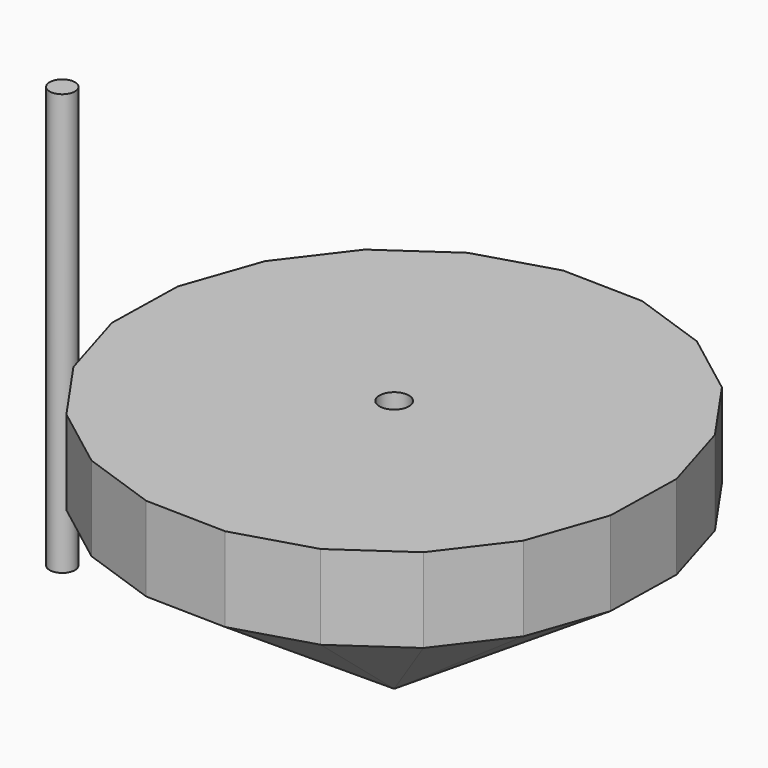
from build123d import *

# Parameters (mm, degrees)
F1_DEPTH     = 30
F2_T1_DEPTH  = 273.0855354784
F2_T3_DEPTH  = 273.0855354784
F2_T5_DEPTH  = 273.0855354784
F2_T7_DEPTH  = 273.0855354784
F2_T9_DEPTH  = 273.0855354784
F2_T11_DEPTH = 273.0855354784
F2_T13_DEPTH = 273.0855354784
F2_T15_DEPTH = 273.0855354784
F2_T17_DEPTH = 273.0855354784
F2_T19_DEPTH = 273.0855354784
F2_T21_DEPTH = 273.0855354784
F2_T23_DEPTH = 273.0855354784
F2_T25_DEPTH = 273.0855354784
F2_T27_DEPTH = 273.0855354784
F2_T29_DEPTH = 273.0855354784
F2_T31_DEPTH = 273.0855354784
F2_T33_DEPTH = 273.0855354784
F2_T35_DEPTH = 273.0855354784
F2_T37_DEPTH = 273.0855354784
F2_T39_DEPTH = 273.0855354784
F3_R         = 1.75
F4_DEPTH     = 24
F5_R         = 1.5
F6_DEPTH     = 50


# Not quite as in the source:
# - a fillet or chamfer that OpenCascade refuses, or shapes differently, is made with other operations: its cross-section is extruded or revolved along the edge and cut away or added


with BuildPart() as f1:
    # F0 (on Top) → F1 (new body)
    with BuildSketch(Plane.XY):
        Polygon((13.2507014279, -27.4548412117), (21.0861784508, -22.0164137096), (26.8575934109, -14.4228662363), (30, -5.4175081257), (30.2057975669, 4.1181534262), (27.4548412117, 13.2507014279), (22.0164137096, 21.0861784508), (14.4228662363, 26.8575934109), (5.4175081257, 30), (-4.1181534262, 30.2057975669), (-13.2507014279, 27.4548412117), (-21.0861784508, 22.0164137096), (-26.8575934109, 14.4228662363), (-30, 5.4175081257), (-30.2057975669, -4.1181534262), (-27.4548412117, -13.2507014279), (-22.0164137096, -21.0861784508), (-14.4228662363, -26.8575934109), (-5.4175081257, -30), (4.1181534262, -30.2057975669), align=None)
    extrude(amount=F1_DEPTH)

    # F2: chamfer of 30 x 20 on 20 edges, made by hand

    # F2_s2 → F2_t1 (cut)
    with BuildSketch(Plane(origin=(-128.9192417481, 44.9861815336, 0), x_dir=(0, 0, 1), z_dir=(0.944167486, -0.3294658683, 0))):
        Polygon((20, 30.1099085987), (0, 0.1099085987), (0, 30.1099085987), align=None)
    extrude(amount=F2_T1_DEPTH, mode=Mode.SUBTRACT)

    # F2_s4 → F2_t3 (cut)
    with BuildSketch(Plane(origin=(-136.5109795463, 2.9461644886, 0), x_dir=(0, 0, 1), z_dir=(0.9997671924, -0.0215768622, 0))):
        Polygon((20, 30.1099085987), (0, 0.1099085987), (0, 30.1099085987), align=None)
    extrude(amount=F2_T3_DEPTH, mode=Mode.SUBTRACT)

    # F2_s6 → F2_t5 (cut)
    with BuildSketch(Plane(origin=(-130.7400715385, -39.3822436636, 0), x_dir=(0, 0, 1), z_dir=(0.9575027202, 0.2884242374, 0))):
        Polygon((20, 30.1099085987), (0, 0.1099085987), (0, 30.1099085987), align=None)
    extrude(amount=F2_T5_DEPTH, mode=Mode.SUBTRACT)

    # F2_s8 → F2_t7 (cut)
    with BuildSketch(Plane(origin=(-39.3822436636, 130.7400715385, 0), x_dir=(0, 0, 1), z_dir=(0.2884242374, -0.9575027202, 0))):
        Polygon((20, 30.1099085987), (0, 0.1099085987), (0, 30.1099085987), align=None)
    extrude(amount=F2_T7_DEPTH, mode=Mode.SUBTRACT)

    # F2_s10 → F2_t9 (cut)
    with BuildSketch(Plane(origin=(-77.8556434138, 112.171414409, 0), x_dir=(0, 0, 1), z_dir=(0.5701923632, -0.8215112105, 0))):
        Polygon((20, 30.1099085987), (0, 0.1099085987), (0, 30.1099085987), align=None)
    extrude(amount=F2_T9_DEPTH, mode=Mode.SUBTRACT)

    # F2_s12 → F2_t11 (cut)
    with BuildSketch(Plane(origin=(-108.7079903345, 82.6226376928, 0), x_dir=(0, 0, 1), z_dir=(0.7961460877, -0.6051044597, 0))):
        Polygon((20, 30.1099085987), (0, 0.1099085987), (0, 30.1099085987), align=None)
    extrude(amount=F2_T11_DEPTH, mode=Mode.SUBTRACT)

    # F2_s14 → F2_t13 (cut)
    with BuildSketch(Plane(origin=(-112.171414409, -77.8556434138, 0), x_dir=(0, 0, 1), z_dir=(0.8215112105, 0.5701923632, 0))):
        Polygon((20, 30.1099085987), (0, 0.1099085987), (0, 30.1099085987), align=None)
    extrude(amount=F2_T13_DEPTH, mode=Mode.SUBTRACT)

    # F2_s16 → F2_t15 (cut)
    with BuildSketch(Plane(origin=(-82.6226376928, -108.7079903345, 0), x_dir=(0, 0, 1), z_dir=(0.6051044597, 0.7961460877, 0))):
        Polygon((20, 30.1099085987), (0, 0.1099085987), (0, 30.1099085987), align=None)
    extrude(amount=F2_T15_DEPTH, mode=Mode.SUBTRACT)

    # F2_s18 → F2_t17 (cut)
    with BuildSketch(Plane(origin=(-44.9861815336, -128.9192417481, 0), x_dir=(0, 0, 1), z_dir=(0.3294658683, 0.944167486, 0))):
        Polygon((20, 30.1099085987), (0, 0.1099085987), (0, 30.1099085987), align=None)
    extrude(amount=F2_T17_DEPTH, mode=Mode.SUBTRACT)

    # F2_s20 → F2_t19 (cut)
    with BuildSketch(Plane(origin=(-2.9461644886, -136.5109795463, 0), x_dir=(0, 0, 1), z_dir=(0.0215768622, 0.9997671924, 0))):
        Polygon((20, 30.1099085987), (0, 0.1099085987), (0, 30.1099085987), align=None)
    extrude(amount=F2_T19_DEPTH, mode=Mode.SUBTRACT)

    # F2_s22 → F2_t21 (cut)
    with BuildSketch(Plane(origin=(39.3822436636, -130.7400715385, 0), x_dir=(0, 0, 1), z_dir=(-0.2884242374, 0.9575027202, 0))):
        Polygon((20, 30.1099085987), (0, 0.1099085987), (0, 30.1099085987), align=None)
    extrude(amount=F2_T21_DEPTH, mode=Mode.SUBTRACT)

    # F2_s24 → F2_t23 (cut)
    with BuildSketch(Plane(origin=(77.8556434138, -112.171414409, 0), x_dir=(0, 0, 1), z_dir=(-0.5701923632, 0.8215112105, 0))):
        Polygon((20, 30.1099085987), (0, 0.1099085987), (0, 30.1099085987), align=None)
    extrude(amount=F2_T23_DEPTH, mode=Mode.SUBTRACT)

    # F2_s26 → F2_t25 (cut)
    with BuildSketch(Plane(origin=(108.7079903345, -82.6226376928, 0), x_dir=(0, 0, 1), z_dir=(-0.7961460877, 0.6051044597, 0))):
        Polygon((20, 30.1099085987), (0, 0.1099085987), (0, 30.1099085987), align=None)
    extrude(amount=F2_T25_DEPTH, mode=Mode.SUBTRACT)

    # F2_s28 → F2_t27 (cut)
    with BuildSketch(Plane(origin=(128.9192417481, -44.9861815336, 0), x_dir=(0, 0, 1), z_dir=(-0.944167486, 0.3294658683, 0))):
        Polygon((20, 30.1099085987), (0, 0.1099085987), (0, 30.1099085987), align=None)
    extrude(amount=F2_T27_DEPTH, mode=Mode.SUBTRACT)

    # F2_s30 → F2_t29 (cut)
    with BuildSketch(Plane(origin=(136.5109795463, -2.9461644886, 0), x_dir=(0, 0, 1), z_dir=(-0.9997671924, 0.0215768622, 0))):
        Polygon((20, 30.1099085987), (0, 0.1099085987), (0, 30.1099085987), align=None)
    extrude(amount=F2_T29_DEPTH, mode=Mode.SUBTRACT)

    # F2_s32 → F2_t31 (cut)
    with BuildSketch(Plane(origin=(130.7400715385, 39.3822436636, 0), x_dir=(0, 0, 1), z_dir=(-0.9575027202, -0.2884242374, 0))):
        Polygon((20, 30.1099085987), (0, 0.1099085987), (0, 30.1099085987), align=None)
    extrude(amount=F2_T31_DEPTH, mode=Mode.SUBTRACT)

    # F2_s34 → F2_t33 (cut)
    with BuildSketch(Plane(origin=(112.171414409, 77.8556434138, 0), x_dir=(0, 0, 1), z_dir=(-0.8215112105, -0.5701923632, 0))):
        Polygon((20, 30.1099085987), (0, 0.1099085987), (0, 30.1099085987), align=None)
    extrude(amount=F2_T33_DEPTH, mode=Mode.SUBTRACT)

    # F2_s36 → F2_t35 (cut)
    with BuildSketch(Plane(origin=(82.6226376928, 108.7079903345, 0), x_dir=(0, 0, 1), z_dir=(-0.6051044597, -0.7961460877, 0))):
        Polygon((20, 30.1099085987), (0, 0.1099085987), (0, 30.1099085987), align=None)
    extrude(amount=F2_T35_DEPTH, mode=Mode.SUBTRACT)

    # F2_s38 → F2_t37 (cut)
    with BuildSketch(Plane(origin=(44.9861815336, 128.9192417481, 0), x_dir=(0, 0, 1), z_dir=(-0.3294658683, -0.944167486, 0))):
        Polygon((20, 30.1099085987), (0, 0.1099085987), (0, 30.1099085987), align=None)
    extrude(amount=F2_T37_DEPTH, mode=Mode.SUBTRACT)

    # F2_s40 → F2_t39 (cut)
    with BuildSketch(Plane(origin=(2.9461644886, 136.5109795463, 0), x_dir=(0, 0, 1), z_dir=(-0.0215768622, -0.9997671924, 0))):
        Polygon((20, 30.1099085987), (0, 0.1099085987), (0, 30.1099085987), align=None)
    extrude(amount=F2_T39_DEPTH, mode=Mode.SUBTRACT)

    # F3 (on face) → F4 (cut)
    with BuildSketch(Plane.XY.offset(30)):
        Circle(F3_R)
    extrude(amount=-F4_DEPTH, mode=Mode.SUBTRACT)


with BuildPart() as f6:
    # F5 (on Top) → F6 (new body)
    with BuildSketch(Plane.XY):
        with Locations((-39.3769755578, 0)):
            Circle(F5_R)
    extrude(amount=F6_DEPTH)


solid = Compound([f1.part, f6.part])
